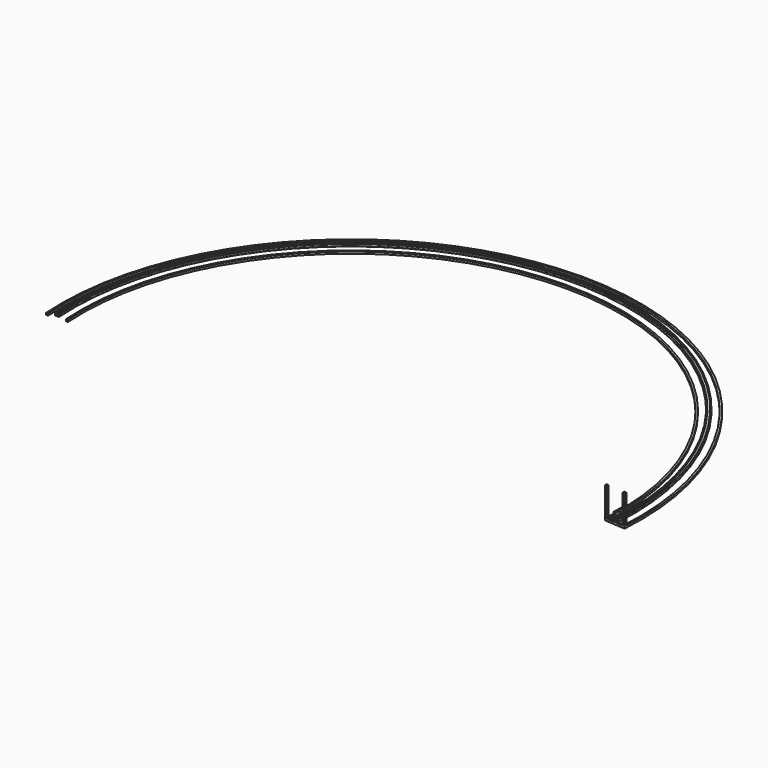
from build123d import *

# Parameters (mm, degrees)
F1_DEPTH = 19.05
F2_W     = 165.1
F2_H     = 19.05
F3_DEPTH = 19.05
F2_W_2   = 19.05
F2_H_2   = 285.75
F8_DEPTH = 15.875


# Not quite as in the source:
# - ends of sketch curves that miss each other by under 0.0002 mm in the source are joined


with BuildPart() as f1:
    # F0 (on Top) → F1 (new body)
    with BuildSketch(Plane.XY):
        with BuildLine():
            Line((2806.6789307259, -189.2186098655), (2825.6857857872, -190.5))
            ThreePointArc((2825.6857857872, -190.5), (0, 2832.1), (-2825.6857857872, -190.5))
            Line((-2825.6857857872, -190.5), (-2806.6789307259, -189.2186098655))
            ThreePointArc((-2806.6789307259, -189.2186098655), (0, 2813.05), (2806.6789307259, -189.2186098655))
        make_face()
    extrude(amount=F1_DEPTH)


with BuildPart() as f1b:
    # F0 (on Top) → F1, piece 2 (new body)
    with BuildSketch(Plane.XY):
        with BuildLine():
            Line((-2641.9528535275, -178.1132286996), (-2622.9459984662, -176.831838565))
            ThreePointArc((-2622.9459984662, -176.831838565), (0, 2628.9), (2622.9459984662, -176.831838565))
            Line((2622.9459984662, -176.831838565), (2641.9528535275, -178.1132286996))
            ThreePointArc((2641.9528535275, -178.1132286996), (0, 2647.95), (-2641.9528535275, -178.1132286996))
        make_face()
    extrude(amount=F1_DEPTH)

    # F7 (on face) → F8 (join)
    with BuildSketch(Plane.XY.offset(19.05)):
        with BuildLine():
            Line((2627.7863839266, -76.5132286996), (2646.8443339823, -76.5132286996))
            Line((2646.8443339823, -76.5132286996), (2646.8623690331, 75.8867702333))
            Line((2646.8623690331, 75.8867702333), (2627.8044192444, 75.8890255555))
            ThreePointArc((2627.8044192444, 75.8890255555), (2628.8999814583, -0.3122318144), (2627.7863839266, -76.5132286996))
        make_face()
    extrude(amount=F8_DEPTH)


with BuildPart() as f3:
    # F2 (on face) → F3 (new body)
    with BuildSketch(Plane(origin=(0, 0, 0), x_dir=(0.9977351738, -0.067264574, 0), z_dir=(-0.067264574, -0.9977351738, 0))):
        with Locations((2730.5, 9.525)):
            Rectangle(F2_W, F2_H)
    extrude(amount=-F3_DEPTH)


with BuildPart() as f3b:
    # F2 (on face) → F3, piece 2 (new body)
    with BuildSketch(Plane(origin=(0, 0, 0), x_dir=(0.9977351738, -0.067264574, 0), z_dir=(-0.067264574, -0.9977351738, 0))):
        with Locations((2638.425, 161.925)):
            Rectangle(F2_W_2, F2_H_2)
    extrude(amount=-F3_DEPTH)


with BuildPart() as f3c:
    # F2 (on face) → F3, piece 3 (new body)
    with BuildSketch(Plane(origin=(0, 0, 0), x_dir=(0.9977351738, -0.067264574, 0), z_dir=(-0.067264574, -0.9977351738, 0))):
        with Locations((2822.575, 161.925)):
            Rectangle(F2_W_2, F2_H_2)
    extrude(amount=-F3_DEPTH)


with BuildPart() as f6:
    # F6: sweep along a path in F4
    with BuildLine(Plane.XY.offset(19.05)) as f6_path:
        ThreePointArc((2724.3158921267, -183.6659192825), (0, 2730.5), (-2724.3158921267, -183.6659192825))
    # F5 (on face) → F6 (sweep)
    with BuildSketch(Plane(origin=(0, 0, 0), x_dir=(0.9977351738, -0.067264574, 0), z_dir=(-0.067264574, -0.9977351738, 0))):
        with BuildLine():
            ThreePointArc((2709.8625, 22.225), (2710.7924359697, 19.9799359697), (2713.0375, 19.05))
            Line((2713.0375, 19.05), (2747.9625, 19.05))
            ThreePointArc((2747.9625, 19.05), (2750.2075640303, 19.9799359697), (2751.1375, 22.225))
            Line((2751.1375, 22.225), (2751.1375, 36.5125))
            ThreePointArc((2751.1375, 36.5125), (2749.7425960454, 39.8800960454), (2746.375, 41.275))
            ThreePointArc((2746.375, 41.275), (2743.0074039546, 39.8800960454), (2741.6125, 36.5125))
            Line((2741.6125, 36.5125), (2741.6125, 34.13125))
            Line((2741.6125, 34.13125), (2744.2795, 34.13125))
            Line((2744.2795, 34.13125), (2744.2795, 36.5125))
            ThreePointArc((2744.2795, 36.5125), (2744.89325774, 37.99424226), (2746.375, 38.608))
            ThreePointArc((2746.375, 38.608), (2747.85674226, 37.99424226), (2748.4705, 36.5125))
            Line((2748.4705, 36.5125), (2748.4705, 22.225))
            ThreePointArc((2748.4705, 22.225), (2748.3217102448, 21.8657897552), (2747.9625, 21.717))
            Line((2747.9625, 21.717), (2713.0375, 21.717))
            ThreePointArc((2713.0375, 21.717), (2712.6782897552, 21.8657897552), (2712.5295, 22.225))
            Line((2712.5295, 22.225), (2712.5295, 36.5125))
            ThreePointArc((2712.5295, 36.5125), (2713.14325774, 37.99424226), (2714.625, 38.608))
            ThreePointArc((2714.625, 38.608), (2716.10674226, 37.99424226), (2716.7205, 36.5125))
            Line((2716.7205, 36.5125), (2716.7205, 34.13125))
            Line((2716.7205, 34.13125), (2719.3875, 34.13125))
            Line((2719.3875, 34.13125), (2719.3875, 36.5125))
            ThreePointArc((2719.3875, 36.5125), (2717.9925960454, 39.8800960454), (2714.625, 41.275))
            ThreePointArc((2714.625, 41.275), (2711.2574039546, 39.8800960454), (2709.8625, 36.5125))
            Line((2709.8625, 36.5125), (2709.8625, 22.225))
        make_face()
    sweep(path=f6_path.line)


solid = Compound([f1.part, f1b.part, f3.part, f3b.part, f3c.part, f6.part])
